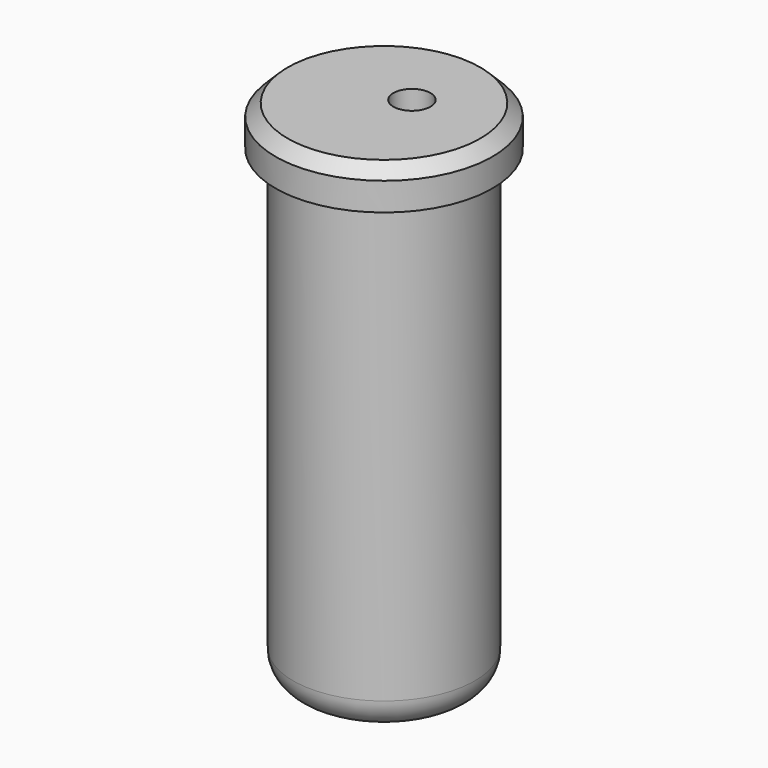
from build123d import *

# Parameters (mm, degrees)
F2_R      = 34.4044739417
F3_DEPTH  = 190.5
F6_R      = 12.7
F8_W      = 45.4750240587
F8_H      = 16.7945176363
F10_R     = 7.7759121847
F11_DEPTH = 177.8
F12_SIZE  = 5.08


# Not quite as in the source:
# - a fillet or chamfer that OpenCascade refuses, or shapes differently, is made with other operations: its cross-section is extruded or revolved along the edge and cut away or added
# - the program builds the solid bodies; features that only make, move or delete a surface that nothing else refers to are left out


with BuildPart() as f1:
    # F0 (on Right) → F1 (revolve)
    with BuildSketch(Plane.YZ):
        Polygon((38.1, -101.6), (38.1, 0), (38.1, 101.6), (0, 101.6), (0, 0), (0, -101.6), align=None)
    revolve(axis=Axis((0, 0, -50.8), (0, 0, -1)))

    # F2 (on face) → F3 (cut)
    with BuildSketch(Plane.XY.offset(101.6)):
        Circle(F2_R)
    extrude(amount=-F3_DEPTH, mode=Mode.SUBTRACT)

    # F6
    f6_edges = [f1.edges().sort_by_distance(p)[0] for p in [
        (0, -38.1, -101.6),
    ]]
    fillet(f6_edges, radius=F6_R)

    # F7: fillet of radius 5.08 on 1 edges, made by hand

    # F7_s1 → F7_t2 (revolve, cut)
    with BuildSketch(Plane.YZ):
        with BuildLine():
            ThreePointArc((38.1, 96.52), (36.6121024484, 100.1121024484), (33.02, 101.6))
            Line((33.02, 101.6), (38.1, 101.6))
            Line((38.1, 101.6), (38.1, 96.52))
        make_face()
    revolve(axis=Axis((0, 0, 101.6), (0, 0, -1)), mode=Mode.SUBTRACT)

    # F8 (on Right) → F9 (revolve)
    with BuildSketch(Plane.YZ):
        with Locations((22.7375120293, 103.7051230669)):
            Rectangle(F8_W, F8_H)
    revolve(axis=Axis((0, 0, 103.7051230669), (0, 0, -1)))

    # F10 (on face) → F11 (cut)
    with BuildSketch(Plane.XY.offset(112.1023818851)):
        with Locations((5.7727694511, 7.4173058383)):
            Circle(F10_R)
    extrude(amount=-F11_DEPTH, mode=Mode.SUBTRACT)

    # F12
    f12_edges = [f1.edges().sort_by_distance(p)[0] for p in [
        (0, -45.475024, 112.102382),
    ]]
    chamfer(f12_edges, length=F12_SIZE)


solid = f1.part
